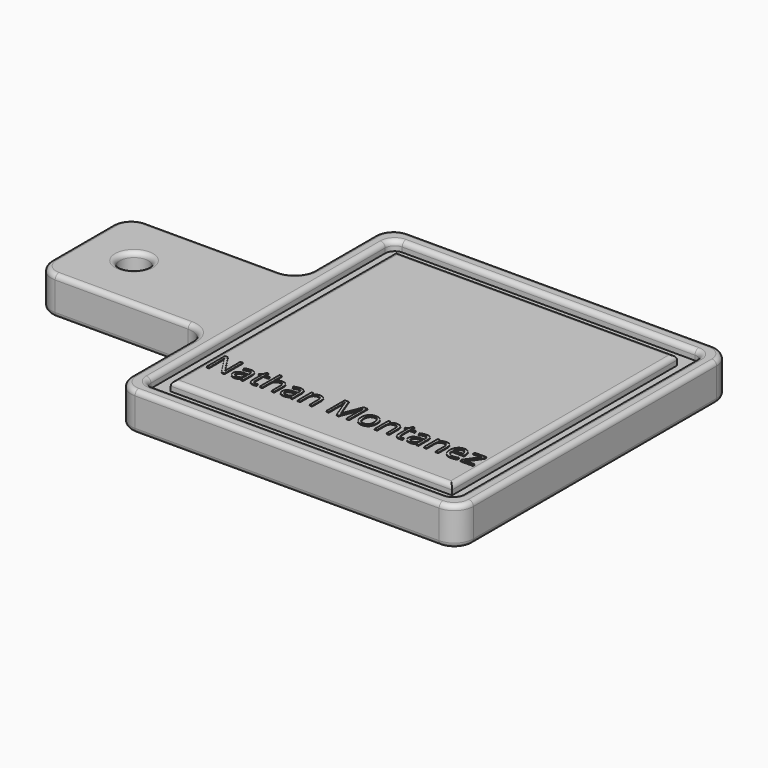
from build123d import *

# Parameters (mm, degrees)
F0_W         = 114.3
F0_H         = 76.2
F1_DEPTH     = 25.4
F2_R         = 9.525
F3_DEPTH     = 25.4
F5_DEPTH     = 6.35
F6_R         = 6.35
F7_R         = 12.7
F8_R         = 3.175
F9_TEXT_SIZE = 21.6097862457
F10_DEPTH    = 0.508


# Not quite as in the source:
# - Text() gives the source's letters only with a copy of the font that has no kerning and outlines rounded to 1/6400 em; it was checked with that copy


with BuildPart() as f1:
    # F0 (on Top) → F1 (new body)
    with BuildSketch(Plane.XY):
        Polygon((0, 76.2), (0, 0), (228.6, 0), (228.6, 228.6), (0, 228.6), (0, 152.4), align=None)
        with Locations((-57.15, 114.3)):
            Rectangle(F0_W, F0_H)
    extrude(amount=F1_DEPTH)

    # F2 (on face) → F3 (cut)
    with BuildSketch(Plane(origin=(0, 0, 0), x_dir=(1, 0, 0), z_dir=(0, 0, -1))):
        with Locations((-79.375, -114.3)):
            Circle(F2_R)
    extrude(amount=-F3_DEPTH, mode=Mode.SUBTRACT)

    # F4 (on face) → F5 (cut)
    with BuildSketch(Plane.XY.offset(25.4)):
        Polygon((10.1600037575, 76.2), (10.1600037575, 10.1600037575), (218.4399962425, 10.1600037575), (218.4399962425, 218.4399962425), (10.1600037575, 218.4399962425), (10.1600037575, 152.4), align=None)
        Polygon((20.3200028896, 76.2), (20.3200028896, 152.4), (20.3200028896, 208.2799971104), (208.2799971104, 208.2799971104), (208.2799971104, 20.3200028896), (20.3200028896, 20.3200028896), align=None, mode=Mode.SUBTRACT)
    extrude(amount=-F5_DEPTH, mode=Mode.SUBTRACT)

    # F6
    f6_edges = [f1.edges().sort_by_distance(p)[0] for p in [
        (10.160004, 218.439996, 22.225),
        (10.160004, 10.160004, 22.225),
        (218.439996, 10.160004, 22.225),
        (218.439996, 218.439996, 22.225),
    ]]
    fillet(f6_edges, radius=F6_R)

    # F7
    f7_edges = [f1.edges().sort_by_distance(p)[0] for p in [
        (0, 0, 12.7),
        (228.6, 0, 12.7),
        (228.6, 228.6, 12.7),
        (0, 228.6, 12.7),
        (0, 152.4, 12.7),
        (-114.3, 152.4, 12.7),
        (-114.3, 76.2, 12.7),
        (0, 76.2, 12.7),
    ]]
    fillet(f7_edges, radius=F7_R)

    # F8
    f8_edges = [f1.edges().sort_by_distance(p)[0] for p in [
        (114.3, 208.279997, 25.4),
        (208.279997, 114.3, 25.4),
        (114.3, 20.320003, 25.4),
        (20.320003, 114.3, 25.4),
        (0, 38.1, 25.4),
        (-3.719744, 72.480256, 25.4),
        (3.719744, 3.719744, 25.4),
        (-57.15, 76.2, 25.4),
        (114.3, 0, 25.4),
        (-110.580256, 79.919744, 25.4),
        (224.880256, 3.719744, 25.4),
        (-114.3, 114.3, 25.4),
        (228.6, 114.3, 25.4),
        (-110.580256, 148.680256, 25.4),
        (224.880256, 224.880256, 25.4),
        (-57.15, 152.4, 25.4),
        (114.3, 228.6, 25.4),
        (-3.719744, 156.119744, 25.4),
        (3.719744, 224.880256, 25.4),
        (0, 190.5, 25.4),
        (114.3, 10.160004, 25.4),
        (12.019876, 12.019876, 25.4),
        (216.580124, 12.019876, 25.4),
        (10.160004, 114.3, 25.4),
        (218.439996, 114.3, 25.4),
        (12.019876, 216.580124, 25.4),
        (216.580124, 216.580124, 25.4),
        (114.3, 218.439996, 25.4),
        (-88.9, 114.3, 25.4),
        (0, 38.1, 0),
        (-3.719744, 72.480256, 0),
        (3.719744, 3.719744, 0),
        (-57.15, 76.2, 0),
        (114.3, 0, 0),
        (-110.580256, 79.919744, 0),
        (224.880256, 3.719744, 0),
        (-114.3, 114.3, 0),
        (228.6, 114.3, 0),
        (-110.580256, 148.680256, 0),
        (224.880256, 224.880256, 0),
        (-57.15, 152.4, 0),
        (114.3, 228.6, 0),
        (-3.719744, 156.119744, 0),
        (3.719744, 224.880256, 0),
        (0, 190.5, 0),
        (-88.9, 114.3, 0),
    ]]
    fillet(f8_edges, radius=F8_R)

    # F9 (on face) → F10 (join)
    with BuildSketch(Plane.XY.offset(25.4)):
        with Locations((23.4950028896, 43.4990790561)):
            Text('Nathan Montanez', F9_TEXT_SIZE, font='Open Sans', text_align=(TextAlign.LEFT, TextAlign.BOTTOM))
    extrude(amount=F10_DEPTH)


solid = f1.part
